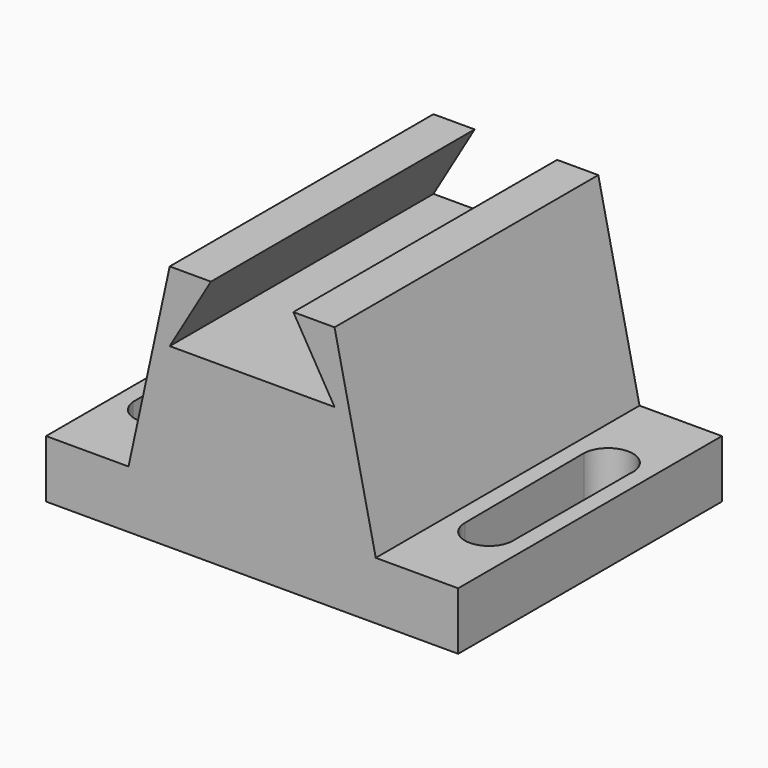
from build123d import *

# Parameters (mm, degrees)
F0_W      = 50
F0_H      = 30
F1_DEPTH  = 40
F2_W      = 10
F2_H      = 23
F3_DEPTH  = 40.001
F5_DEPTH  = 7.001
F7_DEPTH  = 40.001
F8_DEPTH  = 91
F10_DEPTH = 40.001


# Not quite as in the source:
# - an extrude ends at something that could not be found from the text; its depth is read off the source's solid


with BuildPart() as f1:
    # F0 (on Front) → F1 (new body)
    with BuildSketch(Plane.XZ):
        Rectangle(F0_W, F0_H)
    extrude(amount=F1_DEPTH)

    # F2 (on face) → F3 (cut, through all)
    with BuildSketch(Plane.XZ.offset(40)):
        with Locations((-20, 3.5)):
            Rectangle(F2_W, F2_H)
        with Locations((20, 3.5)):
            Rectangle(F2_W, F2_H)
    extrude(amount=-F3_DEPTH, mode=Mode.SUBTRACT)

    # F4 (on face) → F5 (cut, through all)
    with BuildSketch(Plane.XY.offset(-8)):
        with BuildLine():
            Line((-17.1079541888, -29.1274278762), (-16.9848898668, -10.886759475))
            ThreePointArc((-16.9848898668, -10.886759475), (-20.2301216242, -8.0087862495), (-23, -11.346754618))
            Line((-23, -11.346754618), (-22.9528288916, -29.3672662228))
            ThreePointArc((-22.9528288916, -29.3672662228), (-19.9160668858, -32.0334456443), (-17.1079541888, -29.1274278762))
        make_face()
        with BuildLine():
            ThreePointArc((23, -11.346754618), (20.2301216242, -8.0087862495), (16.9848898668, -10.886759475))
            Line((16.9848898668, -10.886759475), (17.1079541888, -29.1274278762))
            ThreePointArc((17.1079541888, -29.1274278762), (19.9160668858, -32.0334456443), (22.9528288916, -29.3672662228))
            Line((22.9528288916, -29.3672662228), (23, -11.346754618))
        make_face()
    extrude(amount=-F5_DEPTH, mode=Mode.SUBTRACT)

    # F6 (on face) → F7 (cut, through all)
    with BuildSketch(Plane.XZ.offset(40)):
        Polygon((15, 15), (10, 15), (15, -8), align=None)
        Polygon((-15, -8), (-10, 15), (-15, 15), align=None)
    extrude(amount=-F7_DEPTH, mode=Mode.SUBTRACT)

    # F6 (on face) → F8 (cut, through all)
    with BuildSketch(Plane.XZ.offset(40)):
        Polygon((-15, -8), (-10, 15), (-15, 15), align=None)
        Polygon((15, 15), (10, 15), (15, -8), align=None)
    extrude(amount=F8_DEPTH, mode=Mode.SUBTRACT)

    # F9 (on face) → F10 (cut, through all)
    with BuildSketch(Plane.XZ.offset(40)):
        Polygon((-5, 15), (-10, 6.486502476), (0, 6.486502476), (10, 6.486502476), (5, 15), align=None)
    extrude(amount=-F10_DEPTH, mode=Mode.SUBTRACT)


solid = f1.part
